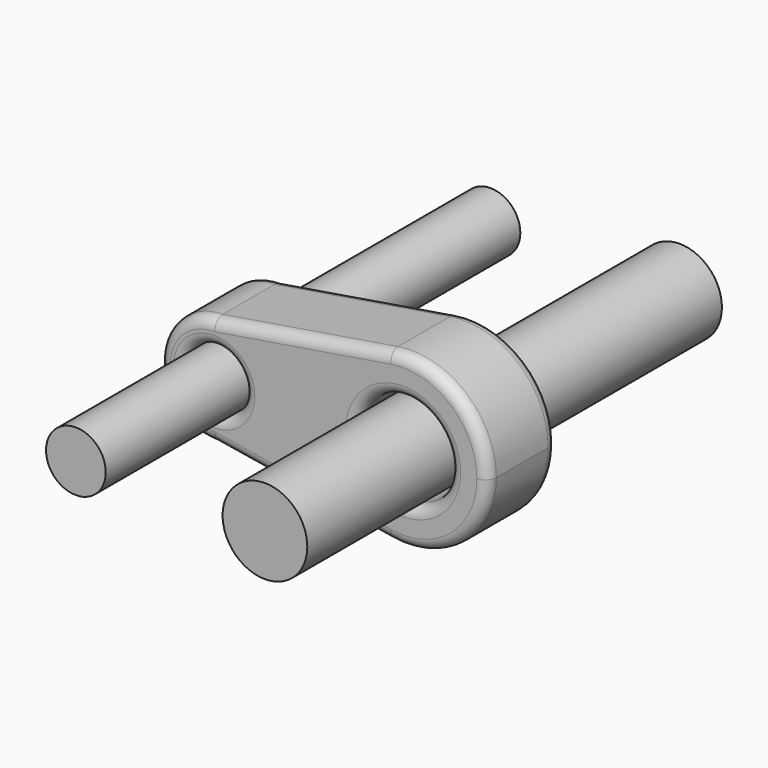
from build123d import *

# Parameters (mm, degrees)
F0_R     = 8.8016886399
F0_R_2   = 13.7313892378
F1_DEPTH = 25.4
F2_R     = 3.17499
F3_R     = 3.175
F4_R     = 8.7766269563
F5_DEPTH = 76.2
F6_R     = 12.4525244068
F7_DEPTH = 76.2


# Not quite as in the source:
# - a fillet or chamfer is up to 0.001 mm smaller than in the source, because OpenCascade refuses the exact size


with BuildPart() as f1:
    # F0 (on Front) → F1 (new body)
    with BuildSketch(Plane.XZ):
        with BuildLine():
            ThreePointArc((0, 16.1029876595), (11.3865317714, 11.3865317714), (16.1029876595, 0))
            ThreePointArc((16.1029876595, 0), (11.3865317714, -11.3865317714), (0, -16.1029876595))
            Line((0, -16.1029876595), (51.5906804684, -24.5315592152))
            ThreePointArc((51.5906804684, -24.5315592152), (30.7417076943, 0), (51.5906804684, 24.5315592152))
            Line((51.5906804684, 24.5315592152), (0, 16.1029876595))
        make_face()
        with BuildLine():
            ThreePointArc((0, -16.1029876595), (11.3865317714, -11.3865317714), (16.1029876595, 0))
            ThreePointArc((16.1029876595, 0), (11.3865317714, 11.3865317714), (0, 16.1029876595))
            ThreePointArc((0, 16.1029876595), (-16.1029876595, 0), (0, -16.1029876595))
        make_face()
        Circle(F0_R, mode=Mode.SUBTRACT)
        with BuildLine():
            ThreePointArc((80.4552870872, 0), (71.6956793123, 18.9404521645), (51.5906804684, 24.5315592152))
            ThreePointArc((51.5906804684, 24.5315592152), (30.7417076943, 0), (51.5906804684, -24.5315592152))
            ThreePointArc((51.5906804684, -24.5315592152), (71.6956793123, -18.9404521645), (80.4552870872, 0))
        make_face()
        with Locations((55.5984973907, 0)):
            Circle(F0_R_2, mode=Mode.SUBTRACT)
    extrude(amount=F1_DEPTH)

    # F2 (radius 3.175 in the source; OpenCascade refuses exactly that, so slightly less here)
    f2_edges = [f1.edges().sort_by_distance(p)[0] for p in [
        (80.455287, 0, 0),
        (25.79534, 0, 20.317273),
        (25.79534, -25.4, 20.317273),
        (25.79534, -25.4, -20.317273),
        (25.79534, 0, -20.317273),
        (80.455287, -25.4, 0),
        (-16.102988, -25.4, 0),
        (-16.102988, 0, 0),
    ]]
    fillet(f2_edges, radius=F2_R)

    # F3
    f3_edges = [f1.edges().sort_by_distance(p)[0] for p in [
        (41.867108, -25.4, 0),
        (-8.801689, -25.4, 0),
        (41.867108, 0, 0),
        (-8.801689, 0, 0),
    ]]
    fillet(f3_edges, radius=F3_R)


with BuildPart() as f5:
    # F4 (on Front) → F5 (new body, symmetric)
    with BuildSketch(Plane.XZ):
        Circle(F4_R)
    extrude(amount=F5_DEPTH, both=True)


with BuildPart() as f7:
    # F6 (on Front) → F7 (new body, symmetric)
    with BuildSketch(Plane.XZ):
        with Locations((55.5984973907, 0)):
            Circle(F6_R)
    extrude(amount=F7_DEPTH, both=True)


solid = Compound([f1.part, f5.part, f7.part])
